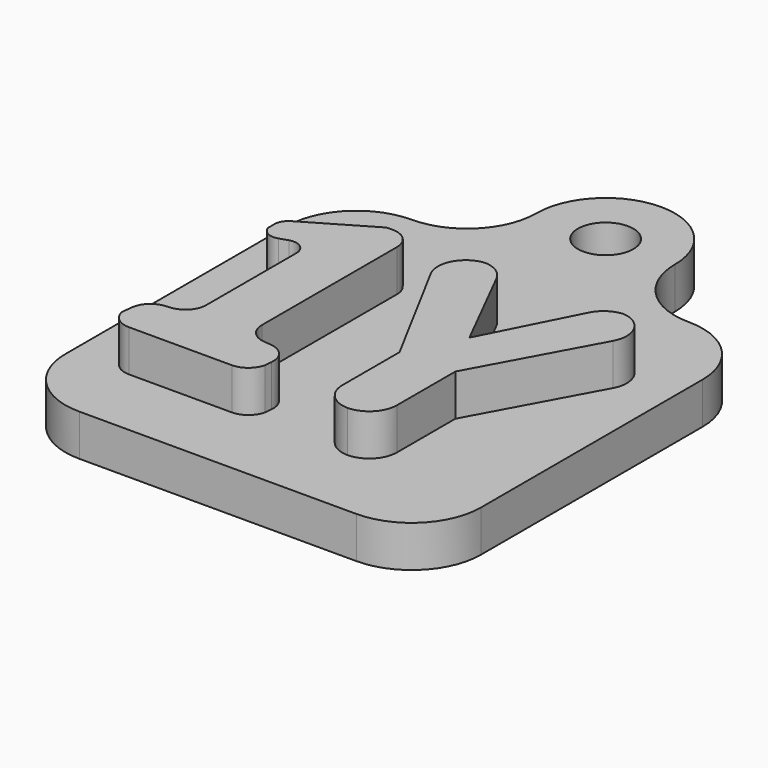
from build123d import *

# Parameters (mm, degrees)
F1_DEPTH       = 3
F2_TEXT_SIZE   = 28.1358076743
F2_TEXT_SIZE_2 = 26.1746536091
F3_DEPTH       = 3
F4_R           = 2
F5_DEPTH       = 6.001
F6_R           = 4.99999
F7_R           = 5
F8_T1_DEPTH    = 8
F8_T3_DEPTH    = 11.4058604216
F8_T5_DEPTH    = 6.0718812943
F8_T7_DEPTH    = 11.3618467234
F8_T9_DEPTH    = 6.0806402078
F9_DEPTH       = 2
F10_DEPTH      = 1
F11_DEPTH      = 1
F12_T1_DEPTH   = 3
F12_T3_DEPTH   = 3
F12_T5_DEPTH   = 6.75
F12_T7_DEPTH   = 6.0481882088
F12_T9_DEPTH   = 6.6650772107
F12_T11_DEPTH  = 6.6650772107
F13_R          = 1.5
F14_R          = 0.99999
F15_R          = 1


# Not quite as in the source:
# - a fillet or chamfer that OpenCascade refuses, or shapes differently, is made with other operations: its cross-section is extruded or revolved along the edge and cut away or added
# - a fillet or chamfer is up to 0.001 mm smaller than in the source, because OpenCascade refuses the exact size
# - Text() gives the source's letters only with a copy of the font that has no kerning and outlines rounded to 1/6400 em; it was checked with that copy


with BuildPart() as f1:
    # F0 (on Top) → F1 (new body)
    with BuildSketch(Plane.XY):
        with BuildLine():
            ThreePointArc((-5, 20), (-3.5355339059, 16.4644660941), (0, 15))
            ThreePointArc((0, 15), (3.5355339059, 16.4644660941), (5, 20))
            ThreePointArc((5, 20), (0, 25), (-5, 20))
        make_face()
        with BuildLine():
            Line((0, 15), (5, 15))
            Line((5, 15), (5, 20))
            ThreePointArc((5, 20), (3.5355339059, 16.4644660941), (0, 15))
        make_face()
        with BuildLine():
            Line((-5, 20), (-5, 15))
            Line((-5, 15), (0, 15))
            ThreePointArc((0, 15), (-3.5355339059, 16.4644660941), (-5, 20))
        make_face()
        Polygon((-15, -15), (15, -15), (15, 15), (5, 15), (0, 15), (-5, 15), (-15, 15), align=None)
    extrude(amount=F1_DEPTH)

    # F2 (on face) → F3 (join)
    with BuildSketch(Plane.XY.offset(3)):
        with Locations((-14.3712430137, -9.7060423737)):
            Text('1', F2_TEXT_SIZE, font='Tinos', font_style=FontStyle.BOLD, text_align=(TextAlign.LEFT, TextAlign.BOTTOM))
        with Locations((-3.0318824629, -9.7060423737)):
            Text('Y', F2_TEXT_SIZE_2, font='Open Sans', font_style=FontStyle.BOLD, text_align=(TextAlign.LEFT, TextAlign.BOTTOM))
    extrude(amount=F3_DEPTH)

    # F4 (on face) → F5 (cut, through all)
    with BuildSketch(Plane(origin=(0, 0, 0), x_dir=(1, 0, 0), z_dir=(0, 0, -1))):
        with Locations((0, -20)):
            Circle(F4_R)
    extrude(amount=-F5_DEPTH, mode=Mode.SUBTRACT)

    # F6 (radius 5 in the source; OpenCascade refuses exactly that, so slightly less here)
    f6_edges = [f1.edges().sort_by_distance(p)[0] for p in [
        (5, 15, 1.5),
        (-5, 15, 1.5),
    ]]
    fillet(f6_edges, radius=F6_R)

    # F7
    f7_edges = [f1.edges().sort_by_distance(p)[0] for p in [
        (-15, 15, 1.5),
        (15, 15, 1.5),
        (-15, -15, 1.5),
        (15, -15, 1.5),
    ]]
    fillet(f7_edges, radius=F7_R)

    # F8: fillet of radius 2 on 6 edges, made by hand

    # F8_s2 → F8_t1 (cut)
    with BuildSketch(Plane.XY.offset(3)):
        with BuildLine():
            ThreePointArc((5.1682386107, -9.7060423737), (3.7540250484, -9.1202559361), (3.1682386107, -7.7060423737))
            Line((3.1682386107, -7.7060423737), (3.1682386107, -9.7060423737))
            Line((3.1682386107, -9.7060423737), (5.1682386107, -9.7060423737))
        make_face()
        with BuildLine():
            ThreePointArc((7.1026162314, -7.7060423737), (6.5168297937, -9.1202559361), (5.1026162314, -9.7060423737))
            Line((5.1026162314, -9.7060423737), (7.1026162314, -9.7060423737))
            Line((7.1026162314, -9.7060423737), (7.1026162314, -7.7060423737))
        make_face()
    extrude(amount=F8_T1_DEPTH, mode=Mode.SUBTRACT)

    # F8_s4 → F8_t3 (cut)
    with BuildSketch(Plane.XY.offset(3)):
        with BuildLine():
            ThreePointArc((9.9403931364, 8.9802064294), (11.6592923414, 8.0026473925), (11.697866095, 6.0255919524))
            Line((11.697866095, 6.0255919524), (13.302737305, 8.9802064294))
            Line((13.302737305, 8.9802064294), (9.9403931364, 8.9802064294))
        make_face()
    extrude(amount=F8_T3_DEPTH, mode=Mode.SUBTRACT)

    # F8_s6 → F8_t5 (cut)
    with BuildSketch(Plane.XY.offset(3)):
        with BuildLine():
            ThreePointArc((8.4776626051, 7.8841058264), (9.2148012196, 8.6842895838), (10.2617494528, 8.9802064294))
            Line((10.2617494528, 8.9802064294), (9.032996935, 8.9802064294))
            Line((9.032996935, 8.9802064294), (8.4776626051, 7.8841058264))
        make_face()
    extrude(amount=F8_T5_DEPTH, mode=Mode.SUBTRACT)

    # F8_s8 → F8_t7 (cut)
    with BuildSketch(Plane.XY.offset(3)):
        with BuildLine():
            ThreePointArc((0.3128562265, 8.9802064294), (-1.403677077, 8.0066144468), (-1.4490073183, 6.0337198476))
            Line((-1.4490073183, 6.0337198476), (-3.0318824629, 8.9802064294))
            Line((-3.0318824629, 8.9802064294), (0.3128562265, 8.9802064294))
        make_face()
    extrude(amount=F8_T7_DEPTH, mode=Mode.SUBTRACT)

    # F8_s10 → F8_t9 (cut)
    with BuildSketch(Plane.XY.offset(3)):
        with BuildLine():
            ThreePointArc((1.8165189172, 7.8795686318), (1.0792534239, 8.6829577919), (0.0301405617, 8.9802064294))
            Line((0.0301405617, 8.9802064294), (1.2623966448, 8.9802064294))
            Line((1.2623966448, 8.9802064294), (1.8165189172, 7.8795686318))
        make_face()
    extrude(amount=F8_T9_DEPTH, mode=Mode.SUBTRACT)

    # F9 (add): faces of the model
    f9_faces = [f1.faces().sort_by_distance(p)[0] for p in [
        (-3.3587120411, -8.3586009593, 4.5),
        (-10.5223524482, -8.3586009593, 4.5),
    ]]
    extrude(f9_faces, amount=F9_DEPTH, dir=(0.1024795785, 0.9947351085, 0))

    # F10 (add): a face of the model
    f10_faces = [f1.faces().sort_by_distance(p)[0] for p in [
        (-4.8564565241, -7.1990076028, 4.5),
    ]]
    extrude(f10_faces, amount=F10_DEPTH)

    # F11 (add): a face of the model
    f11_faces = [f1.faces().sort_by_distance(p)[0] for p in [
        (-10.5157581183, 5.172964044, 4.5),
    ]]
    extrude(f11_faces, amount=F11_DEPTH)

    # F12: fillet of radius 1.5 on 6 edges, made by hand

    # F12_s2 → F12_t1 (join)
    with BuildSketch(Plane.XY.offset(3)):
        with BuildLine():
            ThreePointArc((-3.6126554703, -6.3218536903), (-4.5726189685, -5.8345945349), (-4.9589361026, -4.8297510276))
            Line((-4.9589361026, -4.8297510276), (-4.9589361026, -6.1831571966))
            Line((-4.9589361026, -6.1831571966), (-3.6126554703, -6.3218536903))
        make_face()
    extrude(amount=F12_T1_DEPTH)

    # F12_s4 → F12_t3 (join)
    with BuildSketch(Plane.XY.offset(3)):
        with BuildLine():
            ThreePointArc((-8.9287227167, -4.8726427791), (-9.3148279528, -5.877251387), (-10.27437399, -6.3646804699))
            Line((-10.27437399, -6.3646804699), (-8.9287227167, -6.2254751657))
            Line((-8.9287227167, -6.2254751657), (-8.9287227167, -4.8726427791))
        make_face()
    extrude(amount=F12_T3_DEPTH)

    # F12_s6 → F12_t5 (cut)
    with BuildSketch(Plane.XY.offset(3)):
        with BuildLine():
            ThreePointArc((-1.7072481904, -8.0260916532), (-2.0355789348, -6.9259923818), (-3.0456314854, -6.3802696228))
            Line((-3.0456314854, -6.3802696228), (-1.5535288227, -6.5339889905))
            Line((-1.5535288227, -6.5339889905), (-1.7072481904, -8.0260916532))
        make_face()
    extrude(amount=F12_T5_DEPTH, mode=Mode.SUBTRACT)

    # F12_s8 → F12_t7 (cut)
    with BuildSketch(Plane.XY.offset(3)):
        with BuildLine():
            ThreePointArc((-10.6982199039, -6.4085265989), (-11.60475502, -6.840127836), (-12.0359738399, -7.7468449219))
            Line((-12.0359738399, -7.7468449219), (-11.9110230228, -6.5339889905))
            Line((-11.9110230228, -6.5339889905), (-10.6982199039, -6.4085265989))
        make_face()
    extrude(amount=F12_T7_DEPTH, mode=Mode.SUBTRACT)

    # F12_s10 → F12_t9 (cut)
    with BuildSketch(Plane.XY.offset(3)):
        with BuildLine():
            ThreePointArc((-10.6499512955, -9.7060423737), (-11.5917248217, -9.373545104), (-12.1159821798, -8.5234592074))
            Line((-12.1159821798, -8.5234592074), (-12.1159821798, -9.7060423737))
            Line((-12.1159821798, -9.7060423737), (-10.6499512955, -9.7060423737))
        make_face()
    extrude(amount=F12_T9_DEPTH, mode=Mode.SUBTRACT)

    # F12_s12 → F12_t11 (cut)
    with BuildSketch(Plane.XY.offset(3)):
        with BuildLine():
            ThreePointArc((-1.7584879797, -8.5234592074), (-2.2827453377, -9.373545104), (-3.2245188639, -9.7060423737))
            Line((-3.2245188639, -9.7060423737), (-1.7584879796, -9.7060423737))
            Line((-1.7584879796, -9.7060423737), (-1.7584879797, -8.5234592074))
        make_face()
    extrude(amount=F12_T11_DEPTH, mode=Mode.SUBTRACT)

    # F13
    f13_edges = [f1.edges().sort_by_distance(p)[0] for p in [
        (-4.958936, 8.867987, 4.5),
    ]]
    fillet(f13_edges, radius=F13_R)

    # F14 (radius 1 in the source; OpenCascade refuses exactly that, so slightly less here)
    f14_edges = [f1.edges().sort_by_distance(p)[0] for p in [
        (-11.790912, 3.701891, 4.5),
        (-12.102794, 5.81701, 4.5),
    ]]
    fillet(f14_edges, radius=F14_R)

    # F15
    f15_edges = [f1.edges().sort_by_distance(p)[0] for p in [
        (-8.928723, 4.641418, 4.5),
    ]]
    fillet(f15_edges, radius=F15_R)


solid = f1.part
